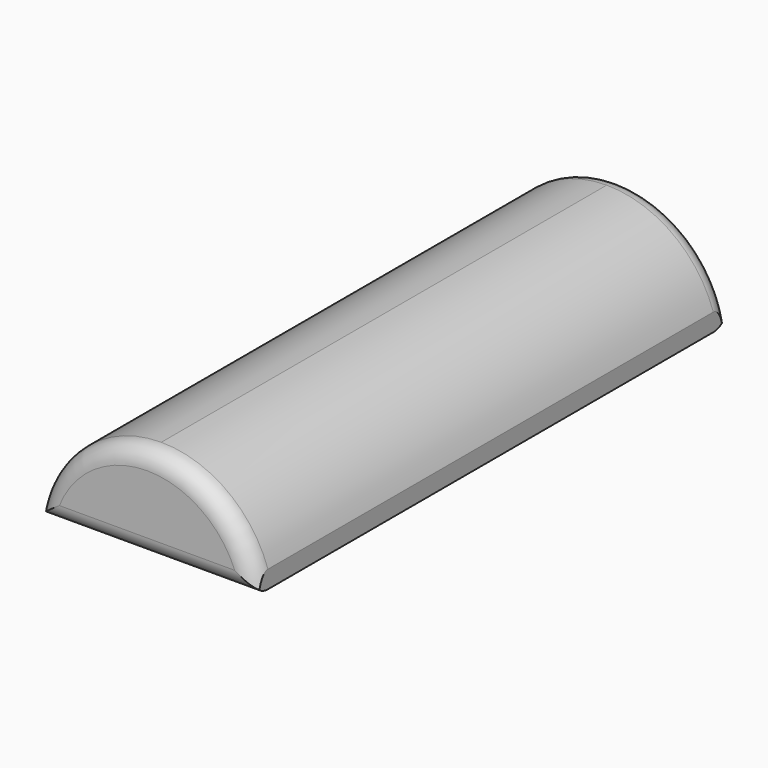
from build123d import *

# Parameters (mm, degrees)
F0_W        = 18
F0_H        = 3
F1_DEPTH    = 100
F2_T1_DEPTH = 51
F2_T4_ANGLE = 188.7220852887
F2_T6_ANGLE = 188.7220852887


# Not quite as in the source:
# - a fillet or chamfer that OpenCascade refuses, or shapes differently, is made with other operations: its cross-section is extruded or revolved along the edge and cut away or added


with BuildPart() as f1:
    # F0 (on Front) → F1 (new body)
    with BuildSketch(Plane.XZ):
        with BuildLine():
            ThreePointArc((0, 9), (-11.1018016556, 5.4101869077), (-18, -4))
            Line((-18, -4), (0, -4))
            Line((0, -4), (0, 0))
            Line((0, 0), (0, 9))
        make_face()
        with BuildLine():
            ThreePointArc((18, -4), (11.1018016556, 5.4101869077), (0, 9))
            Line((0, 9), (0, 0))
            Line((0, 0), (0, -4))
            Line((0, -4), (18, -4))
        make_face()
        with Locations((-9, -5.5)):
            Rectangle(F0_W, F0_H)
        with Locations((9, -5.5)):
            Rectangle(F0_W, F0_H)
    extrude(amount=F1_DEPTH)

    # F2: fillet of radius 3 on 8 edges, made by hand

    # F2_s2 → F2_t1 (cut)
    with BuildSketch(Plane.YZ.offset(-25.5)):
        with BuildLine():
            ThreePointArc((-97, -7), (-99.1213203436, -6.1213203436), (-100, -4))
            Line((-100, -4), (-100, -7))
            Line((-100, -7), (-97, -7))
        make_face()
        with BuildLine():
            ThreePointArc((-3, -7), (-0.8786796564, -6.1213203436), (0, -4))
            Line((0, -4), (0, -7))
            Line((0, -7), (-3, -7))
        make_face()
    extrude(amount=F2_T1_DEPTH, mode=Mode.SUBTRACT)

    # F2_s3 → F2_t4 (revolve, cut)
    with BuildSketch(Plane(origin=(-0.7552929851, 0, -9.9039383967), x_dir=(0, 1, 0), z_dir=(-0.0760410803, 0, -0.9971046856))):
        with BuildLine():
            ThreePointArc((-97, 19.7190246072), (-99.1213203436, 18.8403449507), (-100, 16.7190246072))
            Line((-100, 16.7190246072), (-100, 19.7190246072))
            Line((-100, 19.7190246072), (-97, 19.7190246072))
        make_face()
    revolve(axis=Axis((0, -100, -9.9615384615), (0, -1, 0)), revolution_arc=F2_T4_ANGLE, mode=Mode.SUBTRACT)

    # F2_s5 → F2_t6 (revolve, cut)
    with BuildSketch(Plane(origin=(-0.7552929851, 0, -9.9039383967), x_dir=(0, 1, 0), z_dir=(-0.0760410803, 0, -0.9971046856))):
        with BuildLine():
            ThreePointArc((-3, 19.7190246072), (-0.8786796564, 18.8403449507), (0, 16.7190246072))
            Line((0, 16.7190246072), (0, 19.7190246072))
            Line((0, 19.7190246072), (-3, 19.7190246072))
        make_face()
    revolve(axis=Axis((0, 0, -9.9615384615), (0, -1, 0)), revolution_arc=F2_T6_ANGLE, mode=Mode.SUBTRACT)


solid = f1.part
